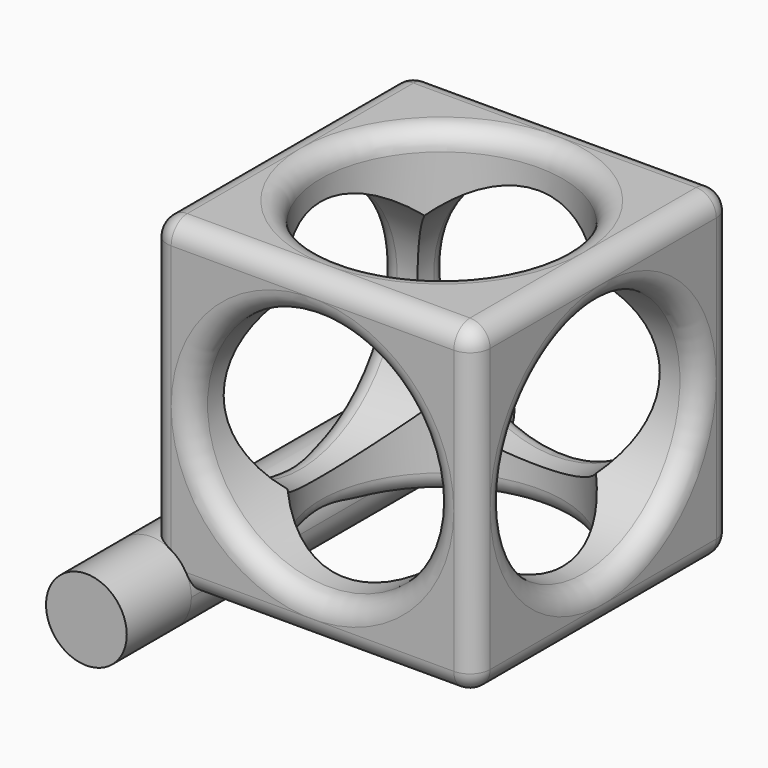
from build123d import *

# Parameters (mm, degrees)
F0_W           = 101.6
F0_H           = 101.6
F1_DEPTH       = 101.6
F2_R           = 38.1
F3_DEPTH       = 101.6
F4_R           = 38.1
F5_DEPTH       = 101.6
F6_R           = 38.1
F7_DEPTH       = 101.6
F8_R           = 6.34999
F10_R          = 12.7
F11_DEPTH      = 25.4
F11_DEPTH_BACK = 127


# Not quite as in the source:
# - a fillet or chamfer is up to 0.001 mm smaller than in the source, because OpenCascade refuses the exact size


with BuildPart() as f1:
    # F0 (on Front) → F1 (new body)
    with BuildSketch(Plane.XZ):
        with Locations((50.8, 50.8)):
            Rectangle(F0_W, F0_H)
    extrude(amount=F1_DEPTH)

    # F2 (on face) → F3 (cut)
    with BuildSketch(Plane.XY.offset(101.6)):
        with Locations((50.8, -50.8)):
            Circle(F2_R)
    extrude(amount=-F3_DEPTH, mode=Mode.SUBTRACT)

    # F4 (on face) → F5 (cut)
    with BuildSketch(Plane(origin=(0, 0, 0), x_dir=(0, -1, 0), z_dir=(-1, 0, 0))):
        with Locations((50.8, 50.8)):
            Circle(F4_R)
    extrude(amount=-F5_DEPTH, mode=Mode.SUBTRACT)

    # F6 (on face) → F7 (cut)
    with BuildSketch(Plane.XZ.offset(101.6)):
        with Locations((50.8, 50.8)):
            Circle(F6_R)
    extrude(amount=-F7_DEPTH, mode=Mode.SUBTRACT)

    # F8 (radius 6.35 in the source; OpenCascade refuses exactly that, so slightly less here)
    f8_edges = [f1.edges().sort_by_distance(p)[0] for p in [
        (101.6, -50.8, 101.6),
        (50.8, 0, 101.6),
        (50.8, -101.6, 101.6),
        (0, -50.8, 101.6),
        (12.7, -50.8, 101.6),
        (0, -101.6, 50.8),
        (50.8, -101.6, 0),
        (101.6, -101.6, 50.8),
        (12.7, -101.6, 50.8),
        (101.6, -50.8, 0),
        (101.6, 0, 50.8),
        (101.6, -12.7, 50.8),
        (0, 0, 50.8),
        (50.8, 0, 0),
        (12.7, 0, 50.8),
        (0, -50.8, 0),
        (0, -12.7, 50.8),
        (12.7, -50.8, 0),
    ]]
    fillet(f8_edges, radius=F8_R)

    # F10 (on offset) → F11 (join, two sides)
    with BuildSketch(Plane.XZ.offset(101.6)) as f11_sk:
        Circle(F10_R)
    extrude(amount=F11_DEPTH)
    extrude(f11_sk.sketch, amount=-F11_DEPTH_BACK)


solid = f1.part
